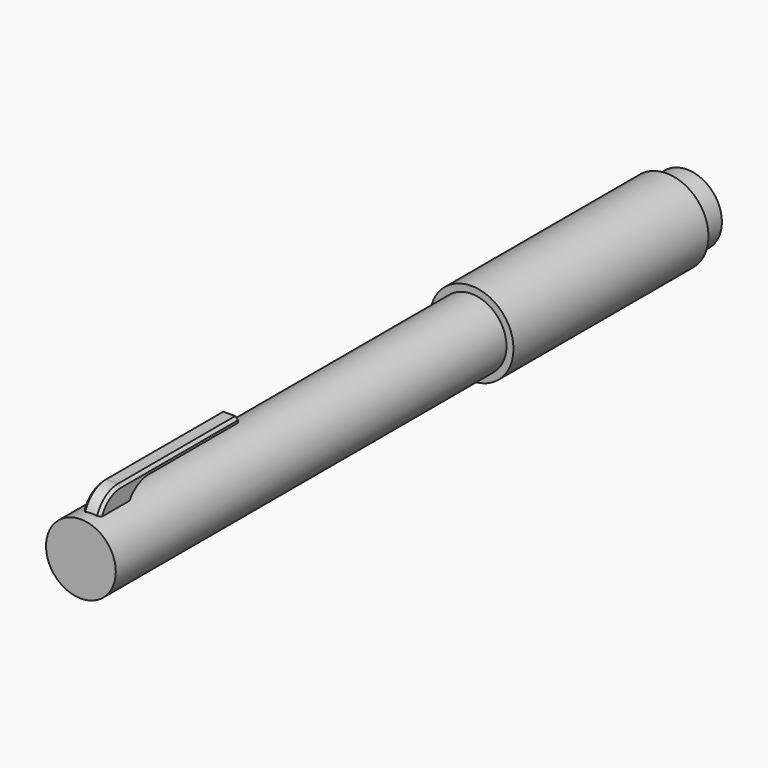
from build123d import *

# Parameters (mm, degrees)
F2_W        = 3.175
F2_H        = 6.35
F3_DEPTH    = 9.525
F4_W        = 3.175
F4_H        = 0.9305988193
F5_DEPTH    = 25.4
F6_R        = 5.08
F7_T1_DEPTH = 27.9764149579
F7_T4_ANGLE = 90
F7_T6_ANGLE = 90
F9_R        = 6.35
F10_DEPTH   = 137.922
F11_R       = 7.62
F12_DEPTH   = 44.3738


# Not quite as in the source:
# - a fillet or chamfer that OpenCascade refuses, or shapes differently, is made with other operations: its cross-section is extruded or revolved along the edge and cut away or added
# - the program builds the solid bodies; features that only make, move or delete a surface that nothing else refers to are left out


with BuildPart() as f3:
    # F2 (on Top) → F3 (new body)
    with BuildSketch(Plane.XY):
        with Locations((0, 5.175651788)):
            Rectangle(F2_W, F2_H)
    extrude(amount=F3_DEPTH)

    # F4 (on face) → F5 (join)
    with BuildSketch(Plane(origin=(0, 8.350651788, 0), x_dir=(-1, 0, 0), z_dir=(0, 1, 0))):
        with Locations((0, 9.0597005904)):
            Rectangle(F4_W, F4_H)
    extrude(amount=F5_DEPTH)

    # F6
    f6_edges = [f3.edges().sort_by_distance(p)[0] for p in [
        (0, 8.350652, 8.594401),
        (0, 2.000652, 9.525),
    ]]
    fillet(f6_edges, radius=F6_R)

    # F7: chamfer of 0.508 on 2 edges, made by hand

    # F7_s2 → F7_t1 (cut)
    with BuildSketch(Plane.XZ.offset(-35.0570667459)):
        Polygon((1.5875, 9.017), (1.0795, 9.525), (1.5875, 9.525), align=None)
        Polygon((-1.5875, 9.017), (-1.0795, 9.525), (-1.5875, 9.525), align=None)
    extrude(amount=F7_T1_DEPTH, mode=Mode.SUBTRACT)

    # F7_s3 → F7_t4 (revolve, cut)
    with BuildSketch(Plane.XZ.offset(-7.080651788)):
        Polygon((-1.5875, 9.017), (-1.0795, 9.525), (-1.5875, 9.525), align=None)
    revolve(axis=Axis((-1.5875, 7.080651788, 4.445), (1, 0, 0)), revolution_arc=F7_T4_ANGLE, mode=Mode.SUBTRACT)

    # F7_s5 → F7_t6 (revolve, cut)
    with BuildSketch(Plane.XZ.offset(-7.080651788)):
        Polygon((1.5875, 9.017), (1.0795, 9.525), (1.5875, 9.525), align=None)
    revolve(axis=Axis((1.5875, 7.080651788, 4.445), (1, 0, 0)), revolution_arc=F7_T6_ANGLE, mode=Mode.SUBTRACT)

    # F9 (on Front) → F10 (join)
    with BuildSketch(Plane.XZ):
        Circle(F9_R)
    extrude(amount=-F10_DEPTH)

    # F11 (on face) → F12 (join)
    with BuildSketch(Plane.XZ.offset(-88.9)):
        Circle(F11_R)
    extrude(amount=-F12_DEPTH)


solid = f3.part
